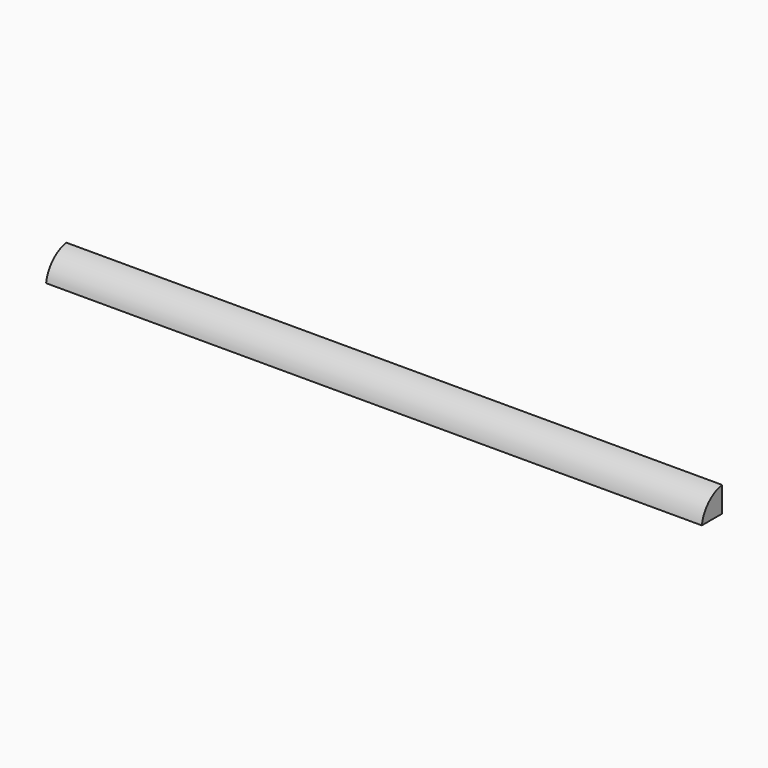
from build123d import *

# Parameters (mm, degrees)
F0_W        = 54.1782
F0_H        = 2.1082
F1_DEPTH    = 2.1082
F2_T1_DEPTH = 66.6933395917


# Not quite as in the source:
# - a fillet or chamfer that OpenCascade refuses, or shapes differently, is made with other operations: its cross-section is extruded or revolved along the edge and cut away or added


with BuildPart() as f1:
    # F0 (on Top) → F1 (new body)
    with BuildSketch(Plane.XY):
        with Locations((27.0891, 1.0541)):
            Rectangle(F0_W, F0_H)
    extrude(amount=F1_DEPTH)

    # F2: fillet of radius 2.54 on 1 edges, made by hand

    # F2_s2 → F2_t1 (cut)
    with BuildSketch(Plane.YZ.offset(-6.2575697959)):
        with BuildLine():
            ThreePointArc((0, -0.3948279183), (0.5972735653, 1.24145262), (2.1082, 2.1082))
            Line((2.1082, 2.1082), (0, 2.1082))
            Line((0, 2.1082), (0, -0.3948279183))
        make_face()
    extrude(amount=F2_T1_DEPTH, mode=Mode.SUBTRACT)


solid = f1.part
